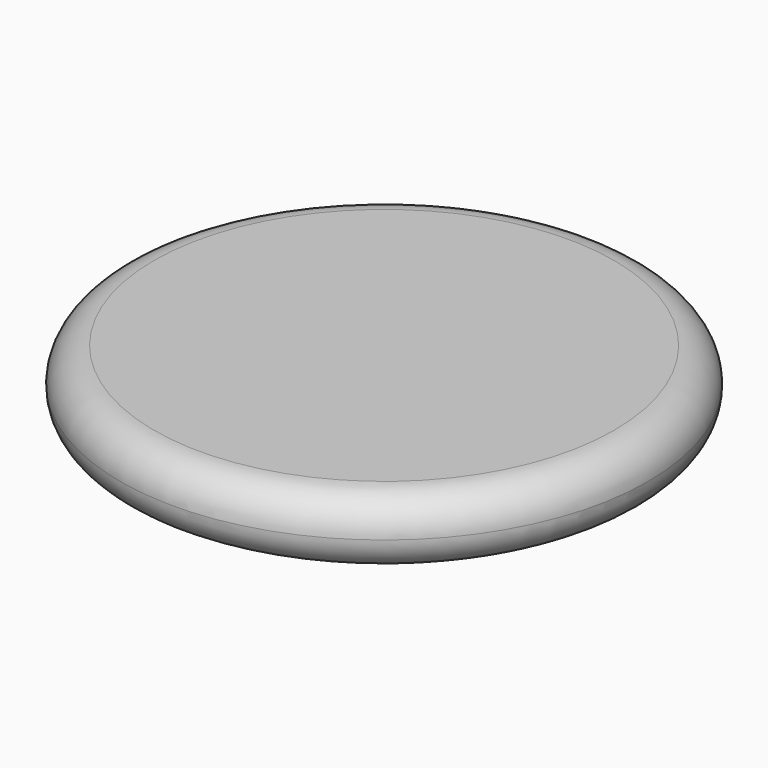
from build123d import *

# Parameters (mm, degrees)
F0_R     = 29.6395356571
F1_DEPTH = 7.62
F2_R     = 3.81
F3_R     = 3.80999


# Not quite as in the source:
# - a fillet or chamfer is up to 0.001 mm smaller than in the source, because OpenCascade refuses the exact size


with BuildPart() as f1:
    # F0 (on Top) → F1 (new body)
    with BuildSketch(Plane.XY):
        Circle(F0_R)
    extrude(amount=F1_DEPTH)

    # F2
    f2_edges = [f1.edges().sort_by_distance(p)[0] for p in [
        (-29.639536, 0, 7.62),
    ]]
    fillet(f2_edges, radius=F2_R)

    # F3 (radius 3.81 in the source; OpenCascade refuses exactly that, so slightly less here)
    f3_edges = [f1.edges().sort_by_distance(p)[0] for p in [
        (-29.639536, 0, 0),
    ]]
    fillet(f3_edges, radius=F3_R)


solid = f1.part
